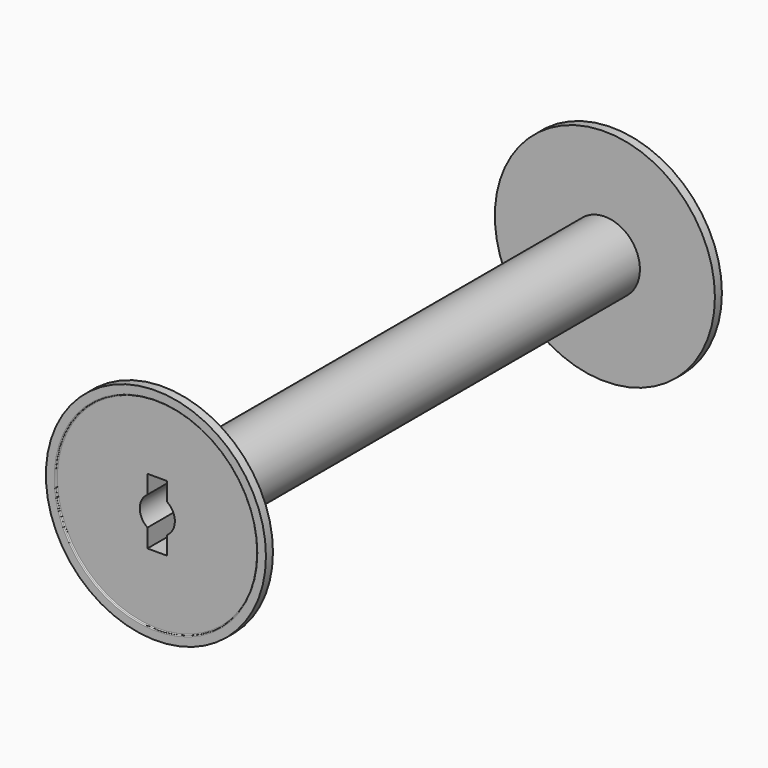
from build123d import *

# Parameters (mm, degrees)
F0_R      = 12.55
F1_DEPTH  = 1
F2_R      = 4
F3_DEPTH  = 63
F4_R      = 12.55
F5_DEPTH  = 1
F6_R      = 11.5
F7_DEPTH  = 0.2
F8_R      = 0.09999
F9_R      = 2
F10_DEPTH = 4
F11_W     = 2.25
F11_H     = 7.5
F12_DEPTH = 5
F13_R     = 11.5
F14_DEPTH = 0.2
F15_R     = 0.09999
F16_R     = 2
F17_DEPTH = 4
F18_W     = 2.25
F18_H     = 7.5
F19_DEPTH = 5


# Not quite as in the source:
# - a fillet or chamfer is up to 0.001 mm smaller than in the source, because OpenCascade refuses the exact size


with BuildPart() as f1:
    # F0 (on Front) → F1 (new body)
    with BuildSketch(Plane.XZ):
        Circle(F0_R)
    extrude(amount=F1_DEPTH)

    # F2 (on face) → F3 (join)
    with BuildSketch(Plane.XZ.offset(1)):
        Circle(F2_R)
    extrude(amount=F3_DEPTH)

    # F4 (on face) → F5 (join)
    with BuildSketch(Plane.XZ.offset(64)):
        Circle(F4_R)
    extrude(amount=F5_DEPTH)

    # F6 (on face) → F7 (cut)
    with BuildSketch(Plane.XZ.offset(65)):
        Circle(F6_R)
    extrude(amount=-F7_DEPTH, mode=Mode.SUBTRACT)

    # F8 (radius 0.1 in the source; OpenCascade refuses exactly that, so slightly less here)
    f8_edges = [f1.edges().sort_by_distance(p)[0] for p in [
        (-11.5, -65, 0),
        (11.5, -64.9, 0),
        (-11.5, -64.8, 0),
    ]]
    fillet(f8_edges, radius=F8_R)

    # F9 (on face) → F10 (cut)
    with BuildSketch(Plane.XZ.offset(64.8)):
        Circle(F9_R)
    extrude(amount=-F10_DEPTH, mode=Mode.SUBTRACT)

    # F11 (on face) → F12 (cut)
    with BuildSketch(Plane(origin=(0, -0.2, 0), x_dir=(-1, 0, 0), z_dir=(0, 1, 0))):
        Rectangle(F11_W, F11_H)
    extrude(amount=-F12_DEPTH, mode=Mode.SUBTRACT)

    # F13 (on face) → F14 (cut)
    with BuildSketch(Plane(origin=(0, 0, 0), x_dir=(-1, 0, 0), z_dir=(0, 1, 0))):
        Circle(F13_R)
    extrude(amount=-F14_DEPTH, mode=Mode.SUBTRACT)

    # F15 (radius 0.1 in the source; OpenCascade refuses exactly that, so slightly less here)
    f15_edges = [f1.edges().sort_by_distance(p)[0] for p in [
        (11.5, 0, 0),
        (11.5, -0.2, 0),
    ]]
    fillet(f15_edges, radius=F15_R)

    # F16 (on face) → F17 (cut)
    with BuildSketch(Plane(origin=(0, -0.2, 0), x_dir=(-1, 0, 0), z_dir=(0, 1, 0))):
        Circle(F16_R)
    extrude(amount=-F17_DEPTH, mode=Mode.SUBTRACT)

    # F18 (on face) → F19 (cut)
    with BuildSketch(Plane.XZ.offset(64.8)):
        Rectangle(F18_W, F18_H)
    extrude(amount=-F19_DEPTH, mode=Mode.SUBTRACT)


solid = f1.part
